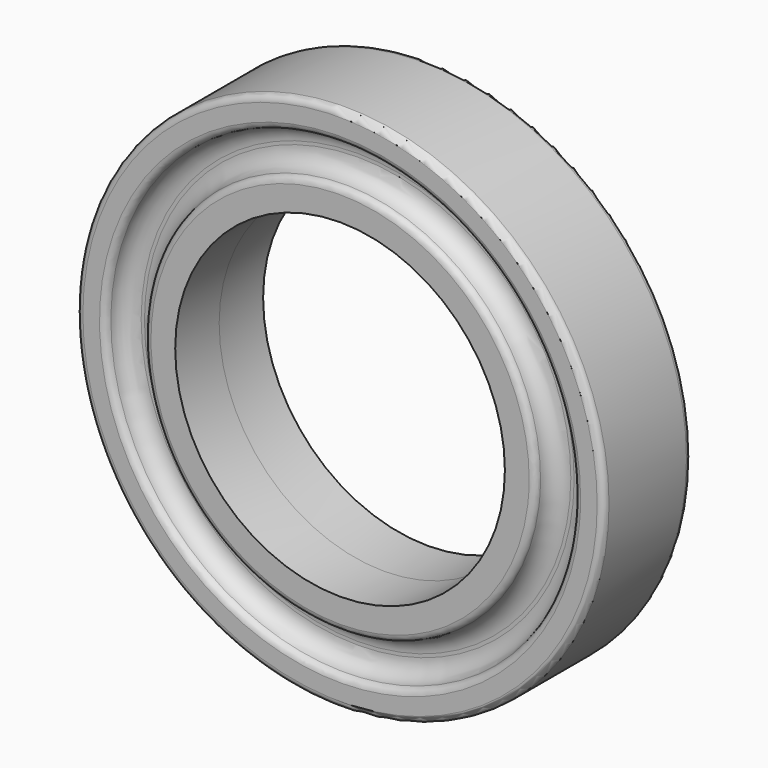
from build123d import *

# Parameters (mm, degrees)
F0_R          = 12
F0_R_2        = 7.5
F1_DEPTH      = 2.5
F1_DEPTH_BACK = 2.5
F2_R          = 10.65
F2_R_2        = 8.9
F3_DEPTH      = 1
F4_R          = 0.8
F5_R          = 0.3


# Not quite as in the source:
# - a pattern or mirror of a feature is missing from the dataset's text; its kind, count and spacing are read off the source's solid


with BuildPart() as f1:
    # F0 (on Front) → F1 (new body, two sides)
    with BuildSketch(Plane.XZ) as f1_sk:
        Circle(F0_R)
        Circle(F0_R_2, mode=Mode.SUBTRACT)
    extrude(amount=F1_DEPTH)
    extrude(f1_sk.sketch, amount=-F1_DEPTH_BACK)

    # F2 (on face) → F3 (cut)
    with BuildSketch(Plane.XZ.offset(2.5)):
        Circle(F2_R)
        Circle(F2_R_2, mode=Mode.SUBTRACT)
    f3 = extrude(amount=-F3_DEPTH, mode=Mode.SUBTRACT)

    # F3_copies: F3 across plane
    add(f3.mirror(Plane.ZX), mode=Mode.SUBTRACT)

    # F4
    f4_edges = [f1.edges().sort_by_distance(p)[0] for p in [
        (-8.9, -1.5, 0),
        (-10.65, -1.5, 0),
        (-10.65, 1.5, 0),
        (-8.9, 1.5, 0),
    ]]
    fillet(f4_edges, radius=F4_R)

    # F5
    f5_edges = [f1.edges().sort_by_distance(p)[0] for p in [
        (-10.65, -2.5, 0),
        (-12, -2.5, 0),
        (-8.9, -2.5, 0),
        (-12, 2.5, 0),
        (-10.65, 2.5, 0),
        (-8.9, 2.5, 0),
    ]]
    fillet(f5_edges, radius=F5_R)


solid = f1.part
